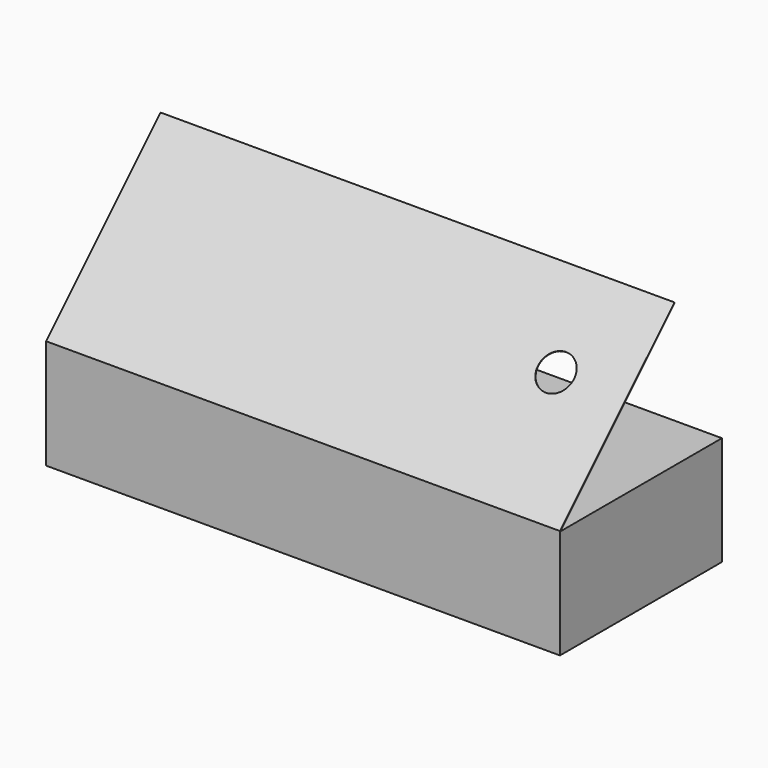
from build123d import *

# Parameters (mm, degrees)
F1_DEPTH = 209.55
F3_DEPTH = 0.4064


# Not quite as in the source:
# - the dataset's text gives a spline's control points without its knots; the knots are read off the source's solid


with BuildPart() as f1:
    # F0 (on Right) → F1 (new body, symmetric)
    with BuildSketch(Plane.YZ):
        Polygon((-165.1, 0), (0, 0), (0, 88.9), (-164.6936, 88.9), (-164.6936, 89.154), (-48.0693022302, 205.7782977698), (-48.3566704261, 206.0656659656), (-165.1, 89.3223363917), align=None)
    extrude(amount=F1_DEPTH, both=True)

    # F2 (on face) → F3 (cut, through all)
    with BuildSketch(Plane(origin=(0, -127.2111681959, 127.2111681959), x_dir=(1, 0, 0), z_dir=(0, -0.7071067812, 0.7071067812))):
        with BuildLine():
            add(Edge.make_bspline(
                [(162.5077574168, 52.5769167773), (159.7895764168, 55.2951231773), (155.9686036168, 56.8776447773), (152.1242374168, 56.8776447773)],
                knots=[7, 7, 7, 7, 8, 8, 8, 8], degree=3))
            add(Edge.make_bspline(
                [(152.1242374168, 56.8776447773), (148.2802014168, 56.8776447773), (144.4592286168, 55.2951231773), (141.7410222168, 52.5769167773)],
                knots=[0, 0, 0, 0, 1, 1, 1, 1], degree=3))
            add(Edge.make_bspline(
                [(141.7410222168, 52.5769167773), (139.0225364168, 49.8585833773), (137.4398624168, 46.0377883773), (137.4398624168, 42.1932697773), (137.4398624168, 38.3492083773), (139.0225364168, 34.5282609773), (141.7410222168, 31.8097497773)],
                knots=[1, 1, 1, 1, 2, 2, 2, 3, 3, 3, 3], degree=3))
            add(Edge.make_bspline(
                [(141.7410222168, 31.8097497773), (144.4592286168, 29.0917211773), (148.2802014168, 27.5088947773), (152.1242374168, 27.5088947773), (155.9686036168, 27.5088947773), (159.7895764168, 29.0917211773), (162.5077574168, 31.8097497773)],
                knots=[3, 3, 3, 3, 4, 4, 4, 5, 5, 5, 5], degree=3))
            add(Edge.make_bspline(
                [(162.5077574168, 31.8097497773), (165.2262686168, 34.5282609773), (166.8086124168, 38.3492083773), (166.8086124168, 42.1932697773), (166.8086124168, 46.0377883773), (165.2262686168, 49.8585833773), (162.5077574168, 52.5769167773)],
                knots=[5, 5, 5, 5, 6, 6, 6, 7, 7, 7, 7], degree=3))
        make_face()
    extrude(amount=-F3_DEPTH, mode=Mode.SUBTRACT)


solid = f1.part
